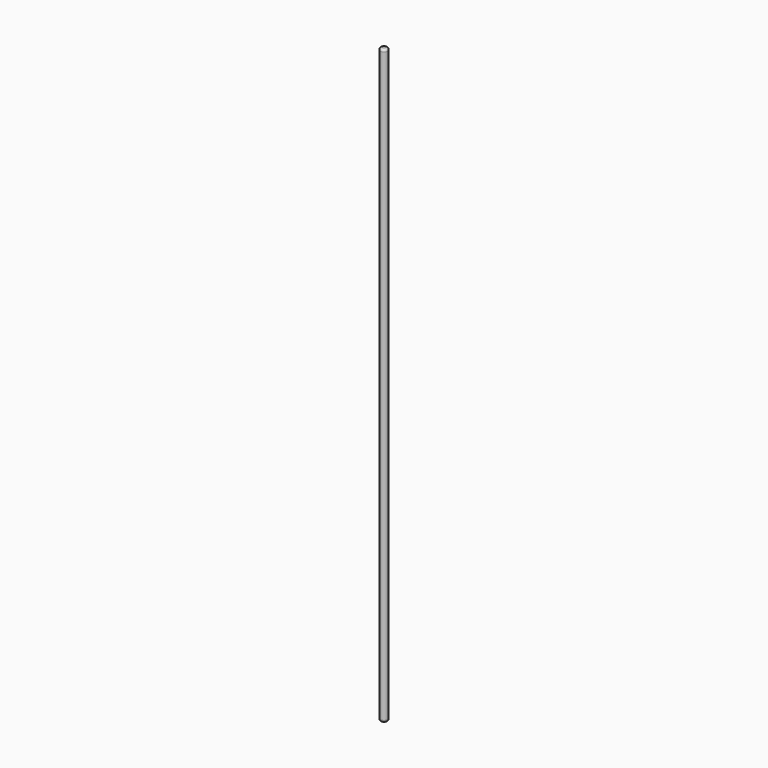
from build123d import *

# Parameters (mm, degrees)
F1_R     = 1.5875
F2_DEPTH = 255
F3_R     = 1


with BuildPart() as f2:
    # F1 (on Top) → F2 (new body)
    with BuildSketch(Plane.XY):
        Circle(F1_R)
    extrude(amount=F2_DEPTH)

    # F3
    f3_edges = [f2.edges().sort_by_distance(p)[0] for p in [
        (-1.5875, 0, 0),
        (-1.5875, 0, 255),
    ]]
    fillet(f3_edges, radius=F3_R)


solid = f2.part
